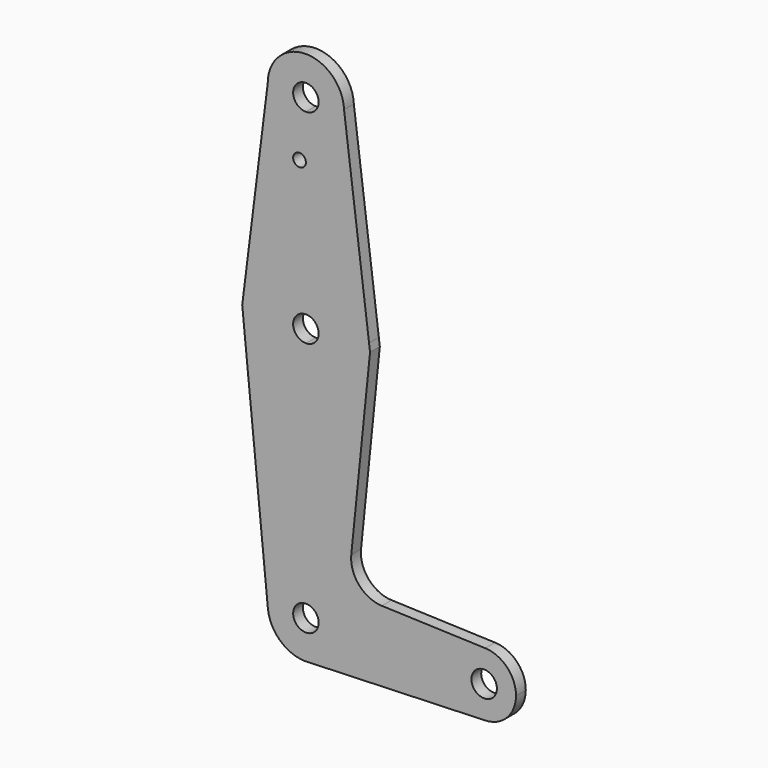
from build123d import *

# Parameters (mm, degrees)
F0_R     = 1.5875
F1_DEPTH = 3.048


with BuildPart() as f1:
    # F0 (on Front) → F1 (new body)
    with BuildSketch(Plane.XZ):
        with BuildLine():
            ThreePointArc((21.1737017489, 108.9369277578), (27.9088938397, 111.726735667), (30.6987017489, 118.4619277578))
            ThreePointArc((30.6987017489, 118.4619277578), (30.6966292861, 118.6606137474), (30.6904127993, 118.8592132763))
            ThreePointArc((30.6904127993, 118.8592132763), (20.9480644341, 127.9842548265), (11.6488543438, 118.4080120008))
            ThreePointArc((11.6488543438, 118.4080120008), (14.4575988085, 111.7077004672), (21.1737017489, 108.9369277578))
        make_face()
        with BuildLine():
            ThreePointArc((24.3487017489, 118.4619277578), (23.4187657792, 116.2168637275), (21.1737017489, 115.2869277578))
            ThreePointArc((21.1737017489, 115.2869277578), (18.9286377187, 120.7069917881), (24.3487017489, 118.4619277578))
        make_face(mode=Mode.SUBTRACT)
        with BuildLine():
            ThreePointArc((30.6904127993, 118.8592132763), (30.6966292861, 118.6606137474), (30.6987017489, 118.4619277578))
            ThreePointArc((30.6987017489, 118.4619277578), (27.9088938397, 111.726735667), (21.1737017489, 108.9369277578))
            Line((21.1737017489, 108.9369277578), (21.1737017489, 104.1871277578))
            Line((21.1737017489, 104.1871277578), (21.1737017489, 83.5369277578))
            ThreePointArc((21.1737017489, 83.5369277578), (31.6700335315, 79.5716987091), (36.9228554319, 69.6568671734))
            Line((36.9228554319, 69.6568671734), (30.6904127993, 118.8592132763))
        make_face()
        with BuildLine():
            Line((21.1737017489, 104.1871277578), (21.1737017489, 108.9369277578))
            ThreePointArc((21.1737017489, 108.9369277578), (14.4575988085, 111.7077004672), (11.6488543438, 118.4080120008))
            Line((11.6488543438, 118.4080120008), (5.7741203481, 71.5178994485))
            ThreePointArc((5.7741203481, 71.5178994485), (11.4063562956, 80.1765027724), (21.1737017489, 83.5369277578))
            Line((21.1737017489, 83.5369277578), (21.1737017489, 104.1871277578))
        make_face()
        with Locations((19.5862017489, 104.1871277578)):
            Circle(F0_R, mode=Mode.SUBTRACT)
        with BuildLine():
            Line((37.1676596329, 67.7242475349), (36.9228554319, 69.6568671734))
            ThreePointArc((36.9228554319, 69.6568671734), (37.0172089319, 68.6613801788), (37.0487017489, 67.6619277578))
            ThreePointArc((37.0487017489, 67.6619277578), (32.3990219003, 56.4366076065), (21.1737017489, 51.7869277578))
            Line((21.1737017489, 51.7869277578), (21.1737017489, 13.6869277578))
            ThreePointArc((21.1737017489, 13.6869277578), (27.9088938397, 10.8971198486), (30.6987017489, 4.1619277578))
            Line((30.6987017489, 4.1619277578), (57.6862017489, 4.1619277578))
            ThreePointArc((57.6862017489, 4.1619277578), (60.1117912642, 9.8735605417), (65.9061070235, 12.0944023724))
            Line((65.9061070235, 12.0944023724), (40.1164770159, 13.0125430406))
            ThreePointArc((40.1164770159, 13.0125430406), (34.4060693237, 15.7340655899), (32.489990471, 21.7626709699))
            Line((32.489990471, 21.7626709699), (37.1676596329, 67.7242475349))
        make_face()
        with BuildLine():
            ThreePointArc((37.0487017489, 67.6619277578), (37.0172089319, 68.6613801788), (36.9228554319, 69.6568671734))
            ThreePointArc((36.9228554319, 69.6568671734), (31.6700335315, 79.5716987091), (21.1737017489, 83.5369277578))
            Line((21.1737017489, 83.5369277578), (21.1737017489, 70.8369277578))
            ThreePointArc((21.1737017489, 70.8369277578), (23.4187657792, 69.9069917881), (24.3487017489, 67.6619277578))
            ThreePointArc((24.3487017489, 67.6619277578), (23.4187657792, 65.4168637275), (21.1737017489, 64.4869277578))
            Line((21.1737017489, 64.4869277578), (21.1737017489, 51.7869277578))
            ThreePointArc((21.1737017489, 51.7869277578), (32.3990219003, 56.4366076065), (37.0487017489, 67.6619277578))
        make_face()
        with BuildLine():
            ThreePointArc((21.1737017489, 83.5369277578), (11.4063562956, 80.1765027724), (5.7741203481, 71.5178994485))
            Line((5.7741203481, 71.5178994485), (5.2988240724, 67.7242475349))
            Line((5.2988240724, 67.7242475349), (5.6202408991, 64.4830159013))
            ThreePointArc((5.6202408991, 64.4830159013), (11.1350165941, 55.3639431521), (21.1737017489, 51.7869277578))
            Line((21.1737017489, 51.7869277578), (21.1737017489, 64.4869277578))
            ThreePointArc((21.1737017489, 64.4869277578), (17.9987017489, 67.6619277578), (21.1737017489, 70.8369277578))
            Line((21.1737017489, 70.8369277578), (21.1737017489, 83.5369277578))
        make_face()
        with BuildLine():
            Line((21.1737017489, 13.6869277578), (21.1737017489, 51.7869277578))
            ThreePointArc((21.1737017489, 51.7869277578), (11.1350165941, 55.3639431521), (5.6202408991, 64.4830159013))
            Line((5.6202408991, 64.4830159013), (11.6951921587, 3.221991086))
            ThreePointArc((11.6951921587, 3.221991086), (14.1140090574, 10.5561723653), (21.1737017489, 13.6869277578))
        make_face()
        with BuildLine():
            ThreePointArc((30.6987017489, 4.1619277578), (27.9088938397, 10.8971198486), (21.1737017489, 13.6869277578))
            Line((21.1737017489, 13.6869277578), (21.1737017489, 7.3369277578))
            ThreePointArc((21.1737017489, 7.3369277578), (23.4187657792, 6.4069917881), (24.3487017489, 4.1619277578))
            Line((24.3487017489, 4.1619277578), (30.6987017489, 4.1619277578))
        make_face()
        with BuildLine():
            Line((21.1737017489, 7.3369277578), (21.1737017489, 13.6869277578))
            ThreePointArc((21.1737017489, 13.6869277578), (14.1140090574, 10.5561723653), (11.6951921587, 3.221991086))
            ThreePointArc((11.6951921587, 3.221991086), (14.6596581325, -2.7873787373), (20.847958208, -5.357500594))
            Line((20.847958208, -5.357500594), (22.168358105, -5.3109959584))
            ThreePointArc((22.168358105, -5.3109959584), (28.2518274469, -2.211906379), (30.6987017489, 4.1619277578))
            Line((30.6987017489, 4.1619277578), (24.3487017489, 4.1619277578))
            ThreePointArc((24.3487017489, 4.1619277578), (18.9286377187, 1.9168637275), (21.1737017489, 7.3369277578))
        make_face()
        with BuildLine():
            Line((57.6862017489, 4.1619277578), (30.6987017489, 4.1619277578))
            ThreePointArc((30.6987017489, 4.1619277578), (28.2518274469, -2.211906379), (22.168358105, -5.3109959584))
            Line((22.168358105, -5.3109959584), (65.9030881784, -3.770653756))
            ThreePointArc((65.9030881784, -3.770653756), (60.1107045393, -1.5486561017), (57.6862017489, 4.1619277578))
        make_face()
        with BuildLine():
            ThreePointArc((73.5612017489, 4.1619277578), (71.3353345329, 9.6738382425), (65.9061070235, 12.0944023724))
            ThreePointArc((65.9061070235, 12.0944023724), (60.1117912642, 9.8735605417), (57.6862017489, 4.1619277578))
            ThreePointArc((57.6862017489, 4.1619277578), (60.1107045393, -1.5486561017), (65.9030881784, -3.770653756))
            ThreePointArc((65.9030881784, -3.770653756), (71.3342856085, -1.3510694518), (73.5612017489, 4.1619277578))
        make_face()
        with BuildLine():
            ThreePointArc((68.7987017489, 4.1619277578), (65.6237017489, 0.9869277578), (62.4487017489, 4.1619277578))
            ThreePointArc((62.4487017489, 4.1619277578), (65.6237017489, 7.3369277578), (68.7987017489, 4.1619277578))
        make_face(mode=Mode.SUBTRACT)
    extrude(amount=F1_DEPTH)


solid = f1.part
